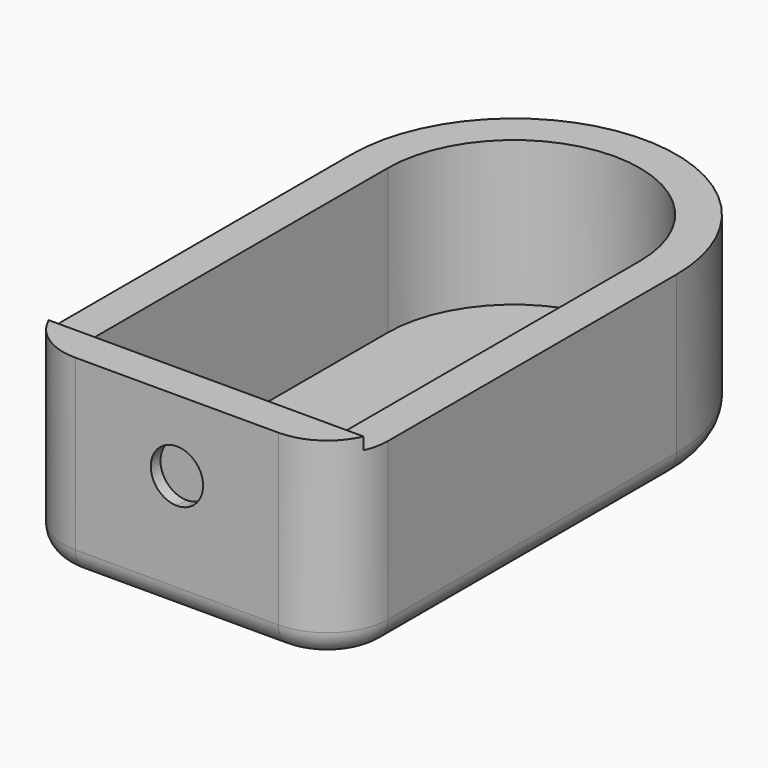
from build123d import *

# Parameters (mm, degrees)
F1_DEPTH    = 3
F2_DEPTH    = 11.9
F4_DEPTH    = 1
F6_DEPTH    = 6
F7_T1_DEPTH = 40.9
F8_R        = 2
F9_R        = 3.5272638361
F10_DEPTH   = 1
F11_DEPTH   = 1


# Not quite as in the source:
# - a fillet or chamfer that OpenCascade refuses, or shapes differently, is made with other operations: its cross-section is extruded or revolved along the edge and cut away or added


with BuildPart() as f1:
    # F0 (on Top) → F1 (new body)
    with BuildSketch(Plane.XY):
        with BuildLine():
            Line((13.35, -34.6), (13.35, 0))
            ThreePointArc((13.35, 0), (0, 13.35), (-13.35, 0))
            Line((-13.35, 0), (-13.35, -34.6))
            Line((-13.35, -34.6), (13.35, -34.6))
        make_face()
        with BuildLine():
            Line((-10.35, -31.6), (-10.35, 0))
            ThreePointArc((-10.35, 0), (0, 10.35), (10.35, 0))
            Line((10.35, 0), (10.35, -31.6))
            Line((10.35, -31.6), (-10.35, -31.6))
        make_face(mode=Mode.SUBTRACT)
        with BuildLine():
            ThreePointArc((10.35, 0), (0, 10.35), (-10.35, 0))
            Line((-10.35, 0), (-10.35, -31.6))
            Line((-10.35, -31.6), (10.35, -31.6))
            Line((10.35, -31.6), (10.35, 0))
        make_face()
    extrude(amount=-F1_DEPTH)

    # F0 (on Top) → F2 (join)
    with BuildSketch(Plane.XY):
        with BuildLine():
            Line((13.35, -34.6), (13.35, 0))
            ThreePointArc((13.35, 0), (0, 13.35), (-13.35, 0))
            Line((-13.35, 0), (-13.35, -34.6))
            Line((-13.35, -34.6), (13.35, -34.6))
        make_face()
        with BuildLine():
            Line((-10.35, -31.6), (-10.35, 0))
            ThreePointArc((-10.35, 0), (0, 10.35), (10.35, 0))
            Line((10.35, 0), (10.35, -31.6))
            Line((10.35, -31.6), (-10.35, -31.6))
        make_face(mode=Mode.SUBTRACT)
    extrude(amount=F2_DEPTH)

    # F3 (on face) → F4 (join)
    with BuildSketch(Plane.XY.offset(11.9)):
        Polygon((-13.35, -34.6), (13.35, -34.6), (13.35, -31.6), (10.35, -31.6), (-10.35, -31.6), (-13.35, -31.6), align=None)
    extrude(amount=F4_DEPTH)

    # F5 (on face) → F6 (cut)
    with BuildSketch(Plane.XZ.offset(34.6)):
        with BuildLine():
            ThreePointArc((0, 9.2), (-2.15, 7.05), (0, 4.9))
            Line((0, 4.9), (0, 9.2))
        make_face()
        with BuildLine():
            Line((0, 9.2), (0, 4.9))
            ThreePointArc((0, 4.9), (1.5202795796, 5.5297204204), (2.15, 7.05))
            ThreePointArc((2.15, 7.05), (1.5202795796, 8.5702795796), (0, 9.2))
        make_face()
    extrude(amount=-F6_DEPTH, mode=Mode.SUBTRACT)

    # F7: fillet of radius 5 on 2 edges, made by hand

    # F7_s2 → F7_t1 (cut)
    with BuildSketch(Plane.XY.offset(-15.5)):
        with BuildLine():
            ThreePointArc((-13.35, -29.6), (-11.8855339059, -33.1355339059), (-8.35, -34.6))
            Line((-8.35, -34.6), (-13.35, -34.6))
            Line((-13.35, -34.6), (-13.35, -29.6))
        make_face()
        with BuildLine():
            ThreePointArc((8.35, -34.6), (11.8855339059, -33.1355339059), (13.35, -29.6))
            Line((13.35, -29.6), (13.35, -34.6))
            Line((13.35, -34.6), (8.35, -34.6))
        make_face()
    extrude(amount=F7_T1_DEPTH, mode=Mode.SUBTRACT)

    # F8
    f8_edges = [f1.edges().sort_by_distance(p)[0] for p in [
        (13.35, -14.8, -3),
    ]]
    fillet(f8_edges, radius=F8_R)

    # F9 (on face) → F10 (join)
    with BuildSketch(Plane(origin=(0, -31.6, 0), x_dir=(-1, 0, 0), z_dir=(0, 1, 0))):
        with Locations((0, 7.05)):
            Circle(F9_R)
    extrude(amount=-F10_DEPTH)

    # F11 (add): a face of the model
    f11_faces = [f1.faces().sort_by_distance(p)[0] for p in [
        (0, -32.6, 7.05),
    ]]
    extrude(f11_faces, amount=F11_DEPTH)


solid = f1.part
